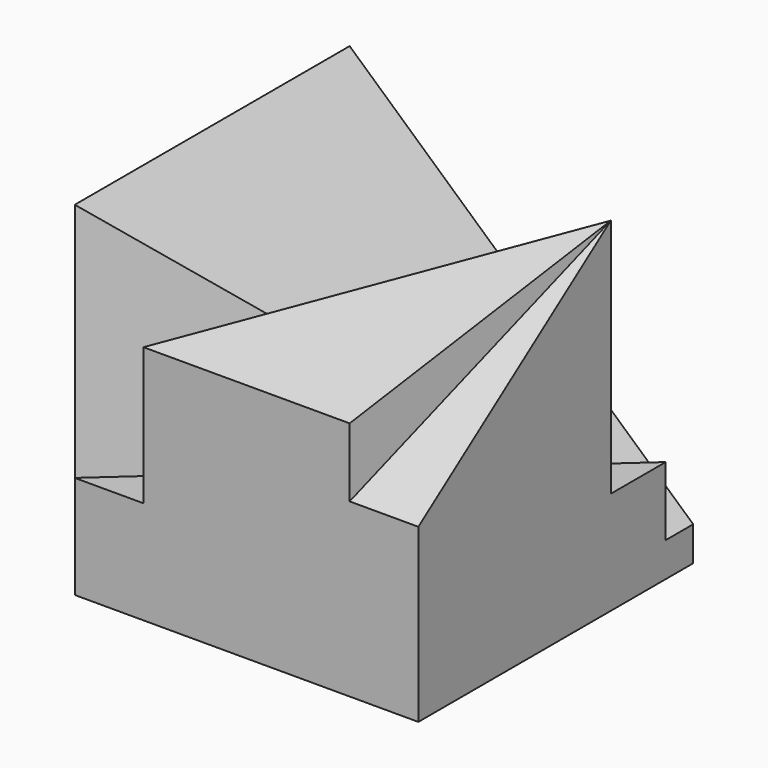
from build123d import *

# Parameters (mm, degrees)
F0_W      = 50
F0_H      = 50
F1_DEPTH  = 50
F4_DEPTH  = 35
F10_REACH = 117.2691203354


with BuildPart() as f1:
    # F0 (on Top) → F1 (new body)
    with BuildSketch(Plane.XY):
        Rectangle(F0_W, F0_H)
    extrude(amount=F1_DEPTH)

    # F3 (on face) → F4 (cut, through all)
    with BuildSketch(Plane.XY.offset(50)):
        Polygon((25, 20), (-25, -25), (-15, -25), (25, 10), align=None)
    extrude(amount=-F4_DEPTH, mode=Mode.SUBTRACT)

    # F5 (on Front) → F6 (revolve, cut)
    with BuildSketch(Plane.XZ):
        Polygon((0, 10), (0, 0), (25, 0), align=None)
    revolve(axis=Axis((0, 0, 5), (0, 0, 1)), mode=Mode.SUBTRACT)

    # F7 (on face) → F8 section 0
    with BuildSketch(Plane.XZ.offset(25), mode=Mode.PRIVATE) as f8_s0:
        Polygon((25, 50), (-15, 50), (-15, 35), (15, 35), (15, 25), (25, 25), align=None)
    loft([f8_s0.sketch, Vertex(25, 10, 50)], mode=Mode.SUBTRACT)

    f10_end = Plane(origin=(0, -2.5, 32.5), x_dir=(-0.7432941462, -0.6689647316, 0), z_dir=(0.6689647316, -0.7432941462, 0))
    # F9 (on face) → F10 (cut, up to a plane its end follows)
    with BuildSketch(Plane(origin=(0, 25, 0), x_dir=(-1, 0, 0), z_dir=(0, 1, 0))):
        Polygon((-25, 5), (25, 50), (-25, 50), align=None)
    f10_long = extrude(amount=-F10_REACH, mode=Mode.PRIVATE)
    add(split(f10_long, bisect_by=f10_end, keep=Keep.BOTTOM, mode=Mode.PRIVATE), mode=Mode.SUBTRACT)


solid = f1.part
